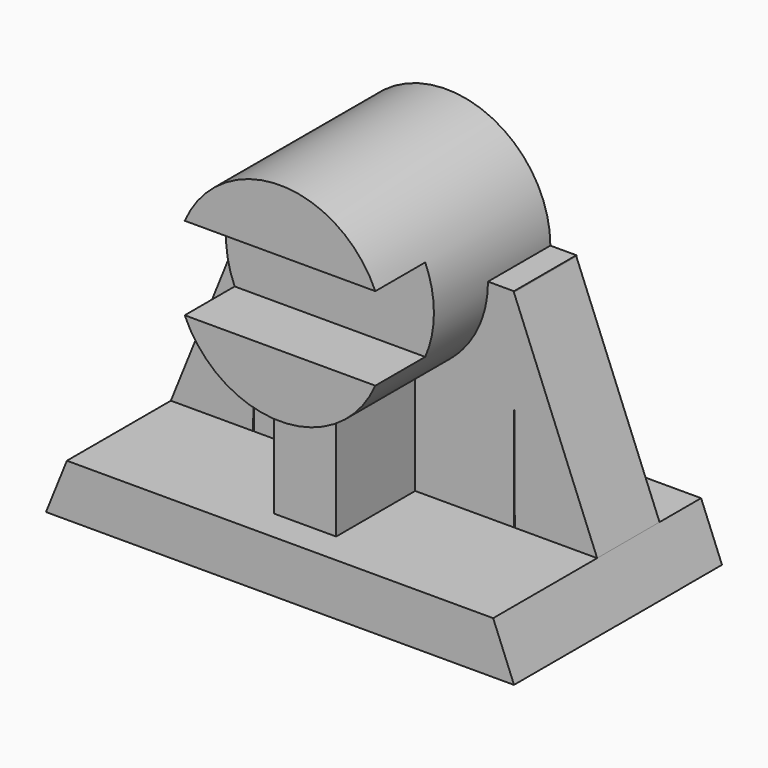
from build123d import *

# Parameters (mm, degrees)
F0_W      = 90
F0_H      = 50
F1_DEPTH  = 10
F2_R      = 20
F3_DEPTH  = 40
F5_DEPTH  = 12
F6_W      = 12
F6_H      = 19
F7_DEPTH  = 25
F9_DEPTH  = 40
F11_DEPTH = 15
F14_DEPTH = 10
F16_DEPTH = 25


with BuildPart() as f1:
    # F0 (on Top) → F1 (new body)
    with BuildSketch(Plane.XY):
        Rectangle(F0_W, F0_H)
    extrude(amount=F1_DEPTH)

    # F6 (on face) → F7 (join)
    with BuildSketch(Plane.XY.offset(10)):
        with Locations((0, -9.5)):
            Rectangle(F6_W, F6_H)
    extrude(amount=F7_DEPTH)

    # F8 (on face) → F9 (join)
    with BuildSketch(Plane.XY.offset(10)):
        Polygon((6, 0), (25, 0), (25, 15), (-25, 15), (-25, 0), (-6, 0), align=None)
    extrude(amount=F9_DEPTH)

    # F10 (on Front) → F11 (join)
    with BuildSketch(Plane.XZ):
        Polygon((-25.21645464, 0), (-24.9451585114, 49.9252006412), (-45.0175479054, 0), align=None)
    extrude(amount=-F11_DEPTH)

    # F12: F1 across plane


with BuildPart() as f3:
    # F2 (on face) → F3 (new body)
    with BuildSketch(Plane.XZ.offset(25)):
        with Locations((0, 50)):
            Circle(F2_R)
    extrude(amount=-F3_DEPTH)

    # F4 (on face) → F5 (cut)
    with BuildSketch(Plane.XZ.offset(25)):
        with BuildLine():
            ThreePointArc((20, 50), (19.5781262586, 45.9138071262), (18.3303027798, 42))
            Line((18.3303027798, 42), (38.403568727, 42))
            Line((38.403568727, 42), (38.403568727, 58))
            Line((38.403568727, 58), (18.3303027798, 58))
            ThreePointArc((18.3303027798, 58), (19.5781262586, 54.0861928738), (20, 50))
        make_face()
        with BuildLine():
            Line((-38.403568727, 58), (-38.403568727, 42))
            Line((-38.403568727, 42), (-18.3303027798, 42))
            ThreePointArc((-18.3303027798, 42), (-20, 50), (-18.3303027798, 58))
            Line((-18.3303027798, 58), (-38.403568727, 58))
        make_face()
        with BuildLine():
            ThreePointArc((-18.3303027798, 58), (-20, 50), (-18.3303027798, 42))
            Line((-18.3303027798, 42), (18.3303027798, 42))
            ThreePointArc((18.3303027798, 42), (19.5781262586, 45.9138071262), (20, 50))
            ThreePointArc((20, 50), (19.5781262586, 54.0861928738), (18.3303027798, 58))
            Line((18.3303027798, 58), (-18.3303027798, 58))
        make_face()
    extrude(amount=-F5_DEPTH, mode=Mode.SUBTRACT)


with BuildPart() as f1_1:
    add(f1.part)
    add(f1.part.mirror(Plane.YZ))

    # F13 (on face) → F14 (cut)
    with BuildSketch(Plane(origin=(-38.7533215674, 0, 15.5807438092), x_dir=(0, -1, 0), z_dir=(-0.9278196121, 0, 0.3730291777))):
        Polygon((33.9928641915, -19.423213931), (33.9928641915, 7.3934104294), (0, 7.3934104294), (0, -6.0149017508), (-15, -6.0149017508), (-15, 7.3934104294), (-48.9928641915, 7.3934104294), (-48.9928641915, -19.423213931), align=None)
    extrude(amount=F14_DEPTH, mode=Mode.SUBTRACT)

    # F15 (on face) → F16 (cut)
    with BuildSketch(Plane(origin=(38.7533215674, 0, 15.5807438092), x_dir=(0, 1, 0), z_dir=(0.9278196121, 0, 0.3730291777))):
        Polygon((0, 9.3338117003), (-31.8076275289, 9.3338117003), (-31.8076275289, -21.363615202), (46.8076275289, -21.363615202), (46.8076275289, 9.3338117003), (15, 9.3338117003), (15, -6.0149017508), (0, -6.0149017508), align=None)
    extrude(amount=F16_DEPTH, mode=Mode.SUBTRACT)


solid = Compound([f3.part, f1_1.part])
